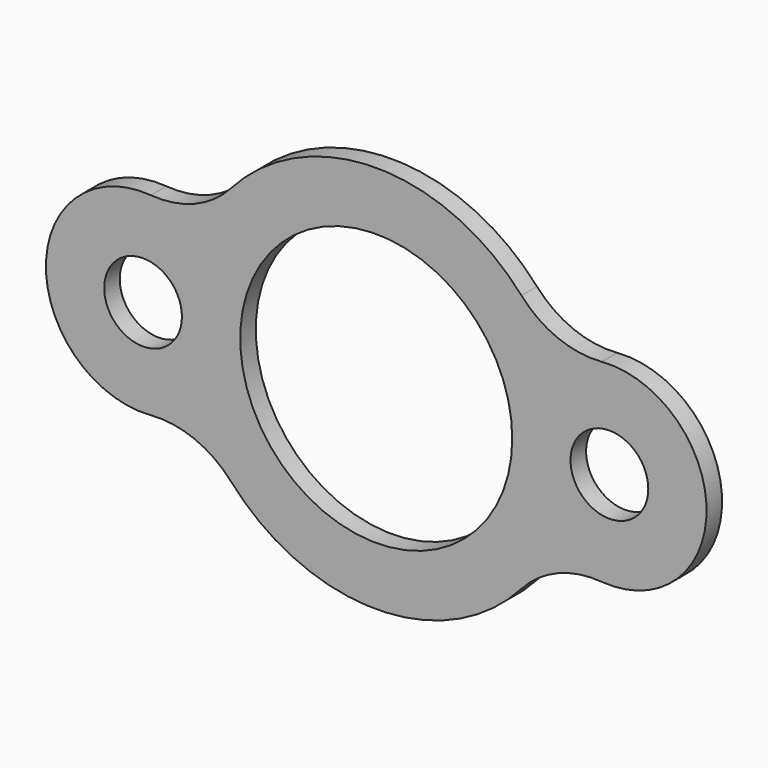
from build123d import *

# Parameters (mm, degrees)
F0_R     = 12.7
F0_R_2   = 44.45
F1_DEPTH = 6.35


# Not quite as in the source:
# - a length typed as a fraction of an inch, garbled in the dataset ("3 / 203.2 mm" for 3/8 in), is restored


with BuildPart() as f1:
    # F0 (on Front) → F1 (new body)
    with BuildSketch(Plane.XZ):
        with BuildLine():
            ThreePointArc((-73.6864583333, -31.6503492602), (-59.3280711503, -33.8428959089), (-47.4486111111, -42.2004656802))
            ThreePointArc((-47.4486111111, -42.2004656802), (0, -63.5), (47.4486111111, -42.2004656802))
            ThreePointArc((47.4486111111, -42.2004656802), (59.3280711503, -33.8428959089), (73.6864583333, -31.6503492602))
            ThreePointArc((73.6864583333, -31.6503492602), (107.95, 0), (73.6864583333, 31.6503492602))
            ThreePointArc((73.6864583333, 31.6503492602), (59.3280711503, 33.8428959089), (47.4486111111, 42.2004656802))
            ThreePointArc((47.4486111111, 42.2004656802), (0, 63.5), (-47.4486111111, 42.2004656802))
            ThreePointArc((-47.4486111111, 42.2004656802), (-59.3280711503, 33.8428959089), (-73.6864583333, 31.6503492602))
            ThreePointArc((-73.6864583333, 31.6503492602), (-107.95, 0), (-73.6864583333, -31.6503492602))
        make_face()
        with Locations((-76.2, 0)):
            Circle(F0_R, mode=Mode.SUBTRACT)
        Circle(F0_R_2, mode=Mode.SUBTRACT)
        with Locations((76.2, 0)):
            Circle(F0_R, mode=Mode.SUBTRACT)
    extrude(amount=F1_DEPTH)


solid = f1.part
